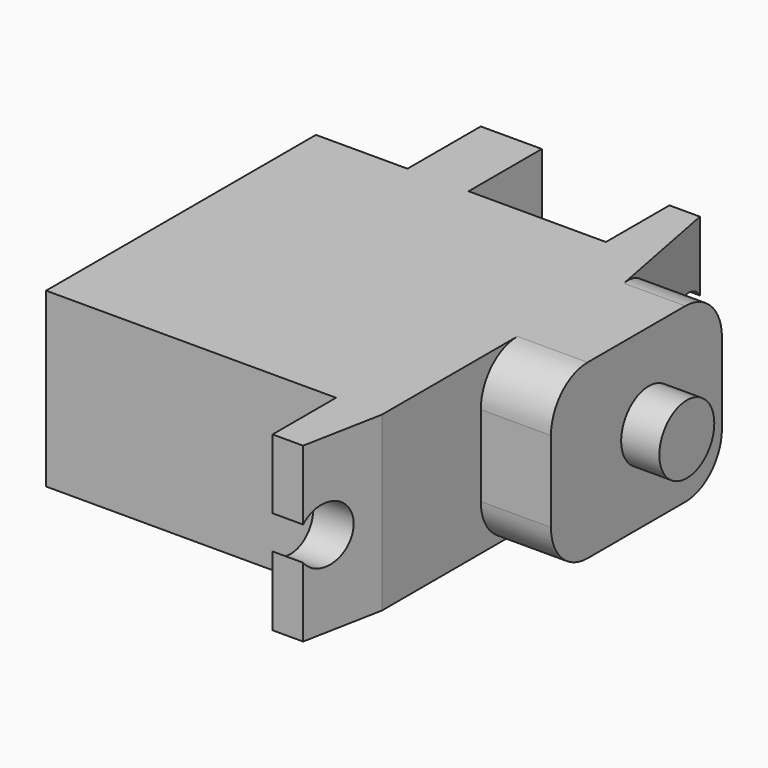
from build123d import *

# Parameters (mm, degrees)
F1_DEPTH = 11.3
F2_R     = 3
F3_R     = 2.25
F4_DEPTH = 2.5
F6_DEPTH = 25


# Not quite as in the source:
# - a feature names something its author has since deleted; it is built from what else it names


with BuildPart() as f1:
    # F0 (on Top) → F1 (new body)
    with BuildSketch(Plane.XY):
        Polygon((0, 22.1), (0, 0), (19, 0), (19, -5.2), (21, -5.2), (22, 0), (22, 8.1), (26.6, 8.1), (26.6, 22.1), (22, 22.1), (21, 27.3), (19, 27.3), (19, 22.1), (10, 22.1), (10, 28.1), (6, 28.1), (6, 22.1), align=None)
    extrude(amount=F1_DEPTH)

    # F2
    f2_edges = [f1.edges().sort_by_distance(p)[0] for p in [
        (24.3, 8.1, 0),
        (24.3, 8.1, 11.3),
        (24.3, 22.1, 11.3),
        (24.3, 22.1, 0),
    ]]
    fillet(f2_edges, radius=F2_R)

    # F3 (on face) → F4 (join)
    with BuildSketch(Plane.YZ.offset(26.6)):
        with Locations((16.1, 5.65)):
            Circle(F3_R)
    extrude(amount=F4_DEPTH)

    # F5 (on face) → F6 (cut)
    with BuildSketch(Plane(origin=(19, 0, 0), x_dir=(0, -1, 0), z_dir=(-1, 0, 0))):
        with BuildLine():
            Line((5.2, 4.55), (5.2, 6.75))
            ThreePointArc((5.2, 6.75), (1.8625525219, 5.65), (5.2, 4.55))
        make_face()
        with BuildLine():
            ThreePointArc((-27.3, 4.55), (-25.2334488328, 3.8929744119), (-23.9625525219, 5.65))
            ThreePointArc((-23.9625525219, 5.65), (-25.2334488328, 7.4070255881), (-27.3, 6.75))
            Line((-27.3, 6.75), (-27.3, 4.55))
        make_face()
    extrude(amount=-F6_DEPTH, mode=Mode.SUBTRACT)


solid = f1.part
